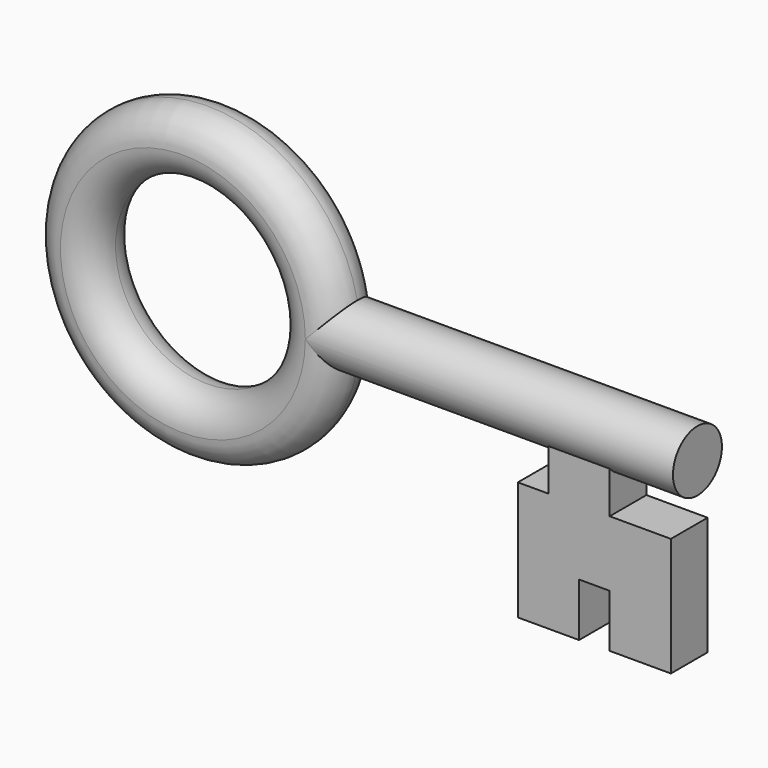
from build123d import *

# Parameters (mm, degrees)
F0_R     = 31.75
F0_R_2   = 19.05
F1_DEPTH = 6.35
F2_R     = 6.34999
F3_R     = 6.34999
F4_W     = 76.2
F4_H     = 6.35
F6_W     = 12.7
F6_H     = 12.7
F6_H_2   = 10.9727999343
F7_DEPTH = 4.7625


# Not quite as in the source:
# - a fillet or chamfer is up to 0.001 mm smaller than in the source, because OpenCascade refuses the exact size


with BuildPart() as f1:
    # F0 (on Front) → F1 (new body, symmetric)
    with BuildSketch(Plane.XZ):
        Circle(F0_R)
        Circle(F0_R_2, mode=Mode.SUBTRACT)
    extrude(amount=F1_DEPTH, both=True)

    # F2 (radius 6.35 in the source; OpenCascade refuses exactly that, so slightly less here)
    f2_edges = [f1.edges().sort_by_distance(p)[0] for p in [
        (-31.75, -6.35, 0),
        (-31.75, 6.35, 0),
    ]]
    fillet(f2_edges, radius=F2_R)

    # F3 (radius 6.35 in the source; OpenCascade refuses exactly that, so slightly less here)
    f3_edges = [f1.edges().sort_by_distance(p)[0] for p in [
        (-19.05, -6.35, 0),
        (-19.05, 6.35, 0),
    ]]
    fillet(f3_edges, radius=F3_R)

    # F4 (on Front) → F5 (revolve)
    with BuildSketch(Plane.XZ):
        with Locations((63.5620742053, 3.175)):
            Rectangle(F4_W, F4_H)
    revolve(axis=Axis((63.5620742053, 0, 0), (1, 0, 0)))

    # F6 (on Front) → F7 (join, symmetric)
    with BuildSketch(Plane.XZ):
        with Locations((80.9154223323, -6.5343625903)):
            Rectangle(F6_W, F6_H)
        Polygon((87.2654223323, -12.8843625903), (74.5654223323, -12.8843625903), (68.2154223323, -12.8843625903), (68.2154223323, -26.4987673753), (74.5654223323, -26.4987673753), (80.9154223323, -26.4987673753), (87.2654223323, -26.4987673753), (99.9654223323, -26.4987673753), (99.9654223323, -12.8843625903), align=None)
        Polygon((74.5654223323, -26.4987673753), (68.2154223323, -26.4987673753), (68.2154223323, -37.5571879506), (80.9154223323, -37.5571879506), (80.9154223323, -26.4987673753), align=None)
        with Locations((93.6154223323, -31.9851673424)):
            Rectangle(F6_W, F6_H_2)
    extrude(amount=F7_DEPTH, both=True)


solid = f1.part
